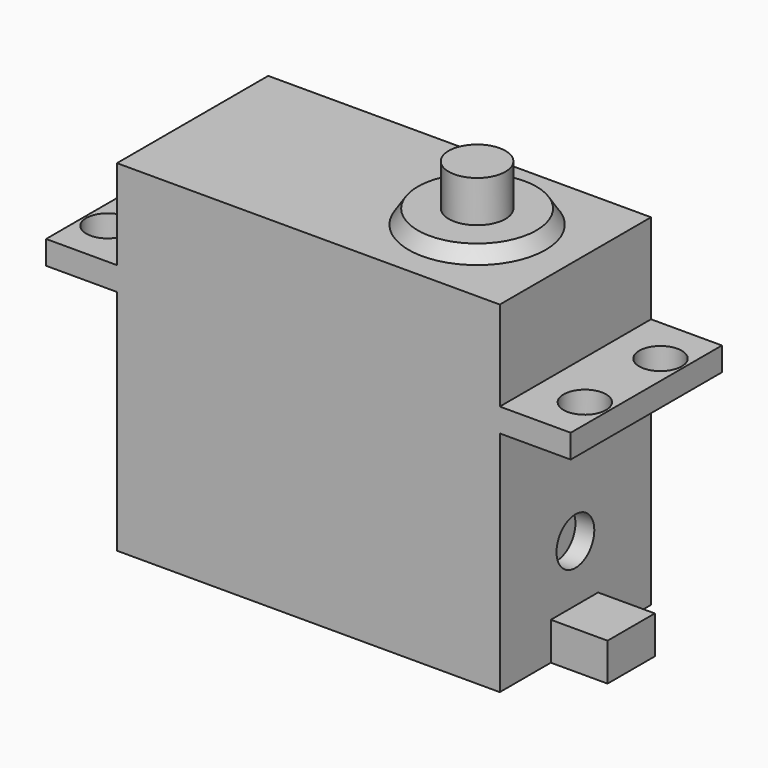
from build123d import *

# Parameters (mm, degrees)
F0_W      = 40.5
F0_H      = 36.1
F1_DEPTH  = 10
F3_W      = 7.5
F3_H      = 20
F3_R      = 2.25
F4_DEPTH  = 2.5
F5_R      = 7.25
F6_DEPTH  = 1.5
F6_TAPER  = 33
F8_R      = 3
F9_DEPTH  = 4.4
F10_R     = 2.5
F11_DEPTH = 2
F12_W     = 6.25
F12_H     = 4
F13_DEPTH = 6


# Not quite as in the source:
# - a feature names something its author has since deleted; it is built from what else it names


with BuildPart() as f1:
    # F0 (on Front) → F1 (new body, symmetric)
    with BuildSketch(Plane.XZ):
        Rectangle(F0_W, F0_H)
    extrude(amount=F1_DEPTH, both=True)

    # F3 (on offset) → F4 (join)
    with BuildSketch(Plane(origin=(0, 0, 8.55), x_dir=(1, 0, 0), z_dir=(0, 0, -1))):
        with Locations((-24, 0)):
            Rectangle(F3_W, F3_H)
        with Locations((-25.25, -5)):
            Circle(F3_R, mode=Mode.SUBTRACT)
        with Locations((-25.25, 5)):
            Circle(F3_R, mode=Mode.SUBTRACT)
        with Locations((24, 0)):
            Rectangle(F3_W, F3_H)
        with Locations((25.25, -5)):
            Circle(F3_R, mode=Mode.SUBTRACT)
        with Locations((25.25, 5)):
            Circle(F3_R, mode=Mode.SUBTRACT)
    extrude(amount=F4_DEPTH)

    # F5 (on face) → F6 (join)
    with BuildSketch(Plane.XY.offset(18.05)):
        with Locations((9.85, 0)):
            Circle(F5_R)
    extrude(amount=F6_DEPTH, taper=F6_TAPER)

    # F8 (on face) → F9 (join, through all)
    with BuildSketch(Plane.XY.offset(19.55)):
        with Locations((9.85, 0)):
            Circle(F8_R)
    extrude(amount=F9_DEPTH)

    # F10 (on face) → F11 (cut)
    with BuildSketch(Plane.YZ.offset(20.25)):
        with Locations((0, -8.05)):
            Circle(F10_R)
    extrude(amount=-F11_DEPTH, mode=Mode.SUBTRACT)

    # F12 (on face) → F13 (join)
    with BuildSketch(Plane.YZ.offset(20.25)):
        with Locations((-0.125, -16.05)):
            Rectangle(F12_W, F12_H)
    extrude(amount=F13_DEPTH)


solid = f1.part
